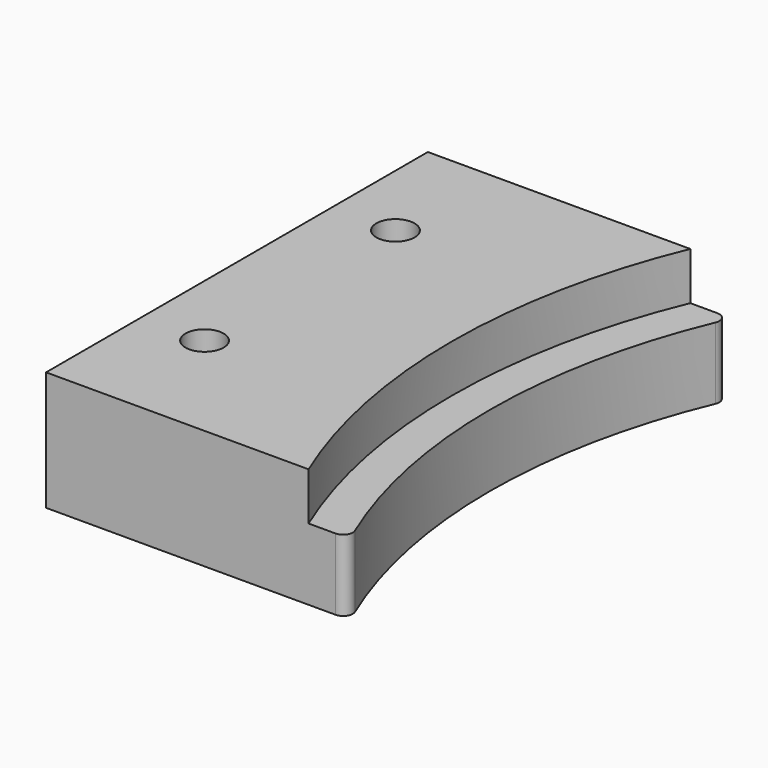
from build123d import *

# Parameters (mm, degrees)
F0_W     = 27.141710973
F0_H     = 25
F0_R     = 2
F2_DEPTH = 25
F1_W     = 8
F1_H     = 10
F4_R     = 1
F5_W     = 175
F5_H     = 25
F6_DEPTH = 25


# Not quite as in the source:
# - a feature names something its author has since deleted; it is built from what else it names


with BuildPart() as f2:
    # F0 (on Top) → F2 (new body)
    with BuildSketch(Plane.XY):
        with BuildLine():
            ThreePointArc((-61, 0), (-59.6453869522, 12.7838888967), (-55.641710973, 25))
            Line((-55.641710973, 25), (-61, 25))
            Line((-61, 25), (-61, 0))
        make_face()
        with BuildLine():
            Line((-59.5, 19.1311264697), (-59.5, 23.5))
            Line((-59.5, 23.5), (-57.9137289423, 23.5))
            ThreePointArc((-57.9137289423, 23.5), (-58.7474910104, 21.3303141089), (-59.5, 19.1311264697))
        make_face(mode=Mode.SUBTRACT)
        with BuildLine():
            ThreePointArc((-55.641710973, -25), (-59.6453869522, -12.7838888967), (-61, 0))
            Line((-61, 0), (-61, -25))
            Line((-61, -25), (-55.641710973, -25))
        make_face()
        with BuildLine():
            Line((-57.9137289423, -23.5), (-59.5, -23.5))
            Line((-59.5, -23.5), (-59.5, -19.1311264697))
            ThreePointArc((-59.5, -19.1311264697), (-58.7474910104, -21.3303141089), (-57.9137289423, -23.5))
        make_face(mode=Mode.SUBTRACT)
        with Locations((-74.5708554865, -12.5)):
            Rectangle(F0_W, F0_H)
        with Locations((-80.891710973, -12.5)):
            Circle(F0_R, mode=Mode.SUBTRACT)
        with Locations((-74.5708554865, 12.5)):
            Rectangle(F0_W, F0_H)
        with Locations((-80.891710973, 12.5)):
            Circle(F0_R, mode=Mode.SUBTRACT)
        with BuildLine():
            Line((-57.9137289423, 23.5), (-59.5, 23.5))
            Line((-59.5, 23.5), (-59.5, 19.1311264697))
            ThreePointArc((-59.5, 19.1311264697), (-58.7474910104, 21.3303141089), (-57.9137289423, 23.5))
        make_face()
        with BuildLine():
            Line((-59.5, -19.1311264697), (-59.5, -23.5))
            Line((-59.5, -23.5), (-57.9137289423, -23.5))
            ThreePointArc((-57.9137289423, -23.5), (-58.7474910104, -21.3303141089), (-59.5, -19.1311264697))
        make_face()
    extrude(amount=F2_DEPTH)

    # F1 (on Front) → F3 (revolve, cut)
    with BuildSketch(Plane.XZ):
        with Locations((-61, 12.5)):
            Rectangle(F1_W, F1_H)
    revolve(axis=Axis((0, 0, 15.2043728158), (0, 0, 1)), mode=Mode.SUBTRACT)

    # F4
    f4_edges = [f2.edges().sort_by_distance(p)[0] for p in [
        (-55.641711, 25, 21.25),
        (-55.641711, 25, 3.75),
        (-55.641711, -25, 3.75),
        (-55.641711, -25, 21.25),
    ]]
    fillet(f4_edges, radius=F4_R)

    # F5 (on Front) → F6 (intersect, symmetric)
    with BuildSketch(Plane.XZ):
        Rectangle(F5_W, F5_H)
    extrude(amount=F6_DEPTH, both=True, mode=Mode.INTERSECT)


solid = f2.part
